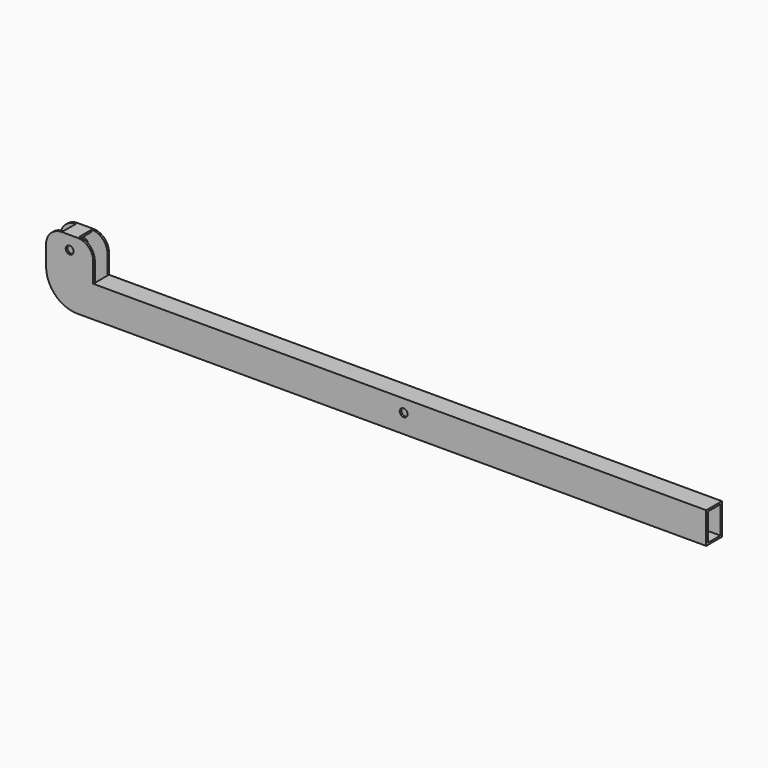
from build123d import *

# Parameters (mm, degrees)
F0_R     = 6.35
F1_DEPTH = 31.75
F2_T     = 3.175


# Not quite as in the source:
# - a shell that OpenCascade refuses in one call is made with other operations: the cavity is built on its own and cut out


with BuildPart() as f1:
    # F0 (on Front) → F1 (new body)
    with BuildSketch(Plane.XZ):
        with BuildLine():
            Line((1066.8, 0), (76.2, 0))
            Line((76.2, 0), (76.2, 31.75))
            ThreePointArc((76.2, 31.75), (68.7605122421, 49.7105122421), (50.8, 57.15))
            Line((50.8, 57.15), (25.4, 57.15))
            ThreePointArc((25.4, 57.15), (7.4394877579, 49.7105122421), (0, 31.75))
            Line((0, 31.75), (0, 0))
            ThreePointArc((0, 0), (14.8789755157, -35.9210244843), (50.8, -50.8))
            Line((50.8, -50.8), (1066.8, -50.8))
            Line((1066.8, -50.8), (1066.8, 0))
        make_face()
        with Locations((577.85, -20.32)):
            Circle(F0_R, mode=Mode.SUBTRACT)
        with Locations((38.1, 35.56)):
            Circle(F0_R, mode=Mode.SUBTRACT)
    extrude(amount=F1_DEPTH)

    # F2: shell of thickness 3.175, made by hand


with BuildPart() as f2_core1:
    # F2_t2: copy of F1
    add(f1.part)

    # the walls: a layer under each face that stays
    f2_faces = [f2_core1.faces().sort_by_distance(p)[0] for p in [
        (571.5, -15.875, 0),
        (38.1, -15.875, 57.15),
        (0, -15.875, 15.875),
        (14.8789755157, -15.875, -35.9210244843),
        (558.8, -15.875, -50.8),
        (177.8, 0, -32.8083333333),
        (177.8, -31.75, -32.8083333333),
    ]]
    thicken(f2_faces, amount=-F2_T, mode=Mode.SUBTRACT)


with BuildPart() as f1_1:
    add(f1.part)

    # what is left inside the walls is the cavity
    f2_cavity = [f2_core1.part.solids().sort_by_distance(p)[0] for p in [
        (533.4, -28.54325, -12.7),
    ]]
    add(f2_cavity, mode=Mode.SUBTRACT)


solid = f1_1.part
